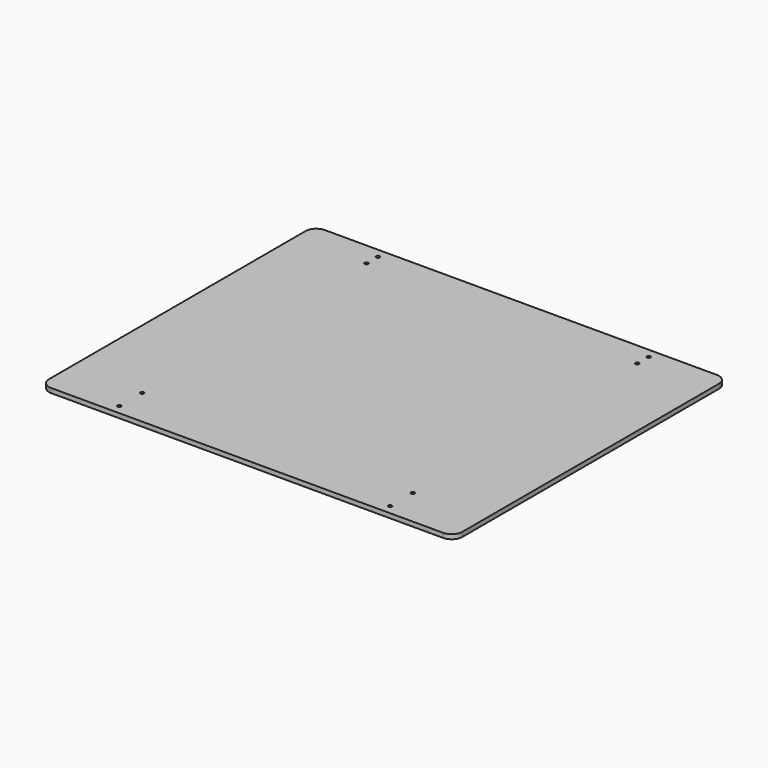
from build123d import *

# Parameters (mm, degrees)
F0_R     = 2.5
F1_DEPTH = 6.35


# Not quite as in the source:
# - a length typed as a fraction of an inch, garbled in the dataset ("3 / 203.2 mm" for 3/8 in), is restored


with BuildPart() as f1:
    # F0 (on Top) → F1 (new body)
    with BuildSketch(Plane.XY):
        with BuildLine():
            Line((-275, -240), (275, -240))
            ThreePointArc((275, -240), (285.6066017178, -235.6066017178), (290, -225))
            Line((290, -225), (290, 225))
            ThreePointArc((290, 225), (285.6066017178, 235.6066017178), (275, 240))
            Line((275, 240), (-275, 240))
            ThreePointArc((-275, 240), (-285.6066017178, 235.6066017178), (-290, 225))
            Line((-290, 225), (-290, -225))
            ThreePointArc((-290, -225), (-285.6066017178, -235.6066017178), (-275, -240))
        make_face()
        with Locations((-190, -226.825)):
            Circle(F0_R, mode=Mode.SUBTRACT)
        with Locations((-190, -186.825)):
            Circle(F0_R, mode=Mode.SUBTRACT)
        with Locations((190, -226.825)):
            Circle(F0_R, mode=Mode.SUBTRACT)
        with Locations((190, -186.825)):
            Circle(F0_R, mode=Mode.SUBTRACT)
        with Locations((-190, 206.825)):
            Circle(F0_R, mode=Mode.SUBTRACT)
        with Locations((-190, 226.825)):
            Circle(F0_R, mode=Mode.SUBTRACT)
        with BuildLine():
            ThreePointArc((190, 209.325), (191.767766953, 208.592766953), (192.5, 206.825))
            ThreePointArc((192.5, 206.825), (188.232233047, 205.057233047), (190, 209.325))
        make_face(mode=Mode.SUBTRACT)
        with BuildLine():
            ThreePointArc((192.5, 226.825), (191.767766953, 225.057233047), (190, 224.325))
            ThreePointArc((190, 224.325), (188.232233047, 228.592766953), (192.5, 226.825))
        make_face(mode=Mode.SUBTRACT)
    extrude(amount=-F1_DEPTH)


solid = f1.part
